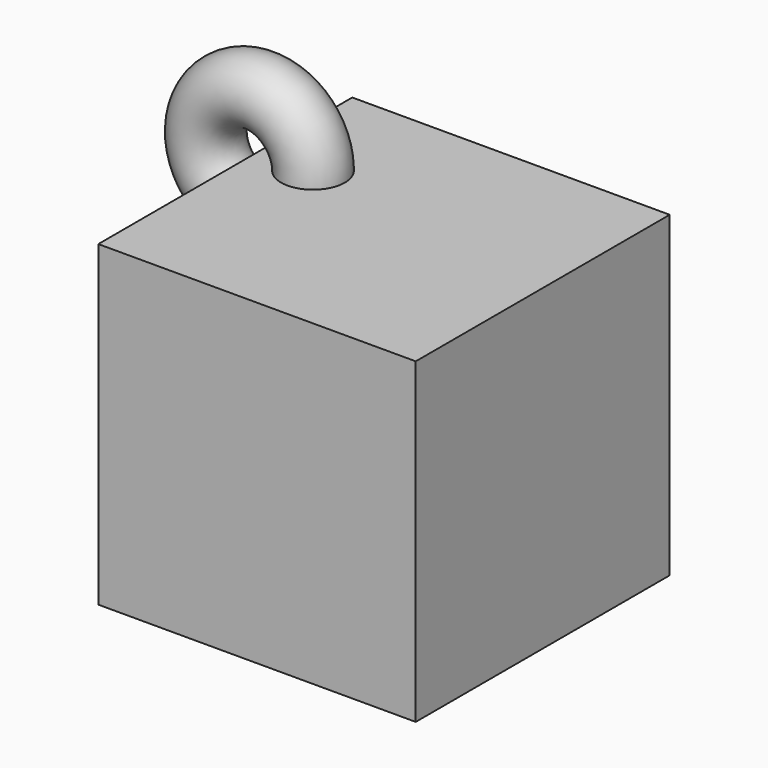
from build123d import *

# Parameters (mm, degrees)
F0_W     = 76.2
F0_H     = 76.2
F1_DEPTH = 76.2
F5_R     = 7.6683459061


# Not quite as in the source:
# - the program builds the solid bodies; features that only make, move or delete a surface that nothing else refers to are left out


with BuildPart() as f1:
    # F0 (on Front) → F1 (new body)
    with BuildSketch(Plane.XZ):
        with Locations((38.1, 38.1)):
            Rectangle(F0_W, F0_H)
    extrude(amount=F1_DEPTH)


with BuildPart() as f6:
    # F5 (on face) → F6 (revolve)
    with BuildSketch(Plane(origin=(0, 0, 0), x_dir=(0, -1, 0), z_dir=(-1, 0, 0))):
        with Locations((27.8481394053, 63.3231475949)):
            Circle(F5_R)
    revolve(axis=Axis((0, -38.1, 76.2), (0, 1, 0)))


solid = Compound([f1.part, f6.part])
